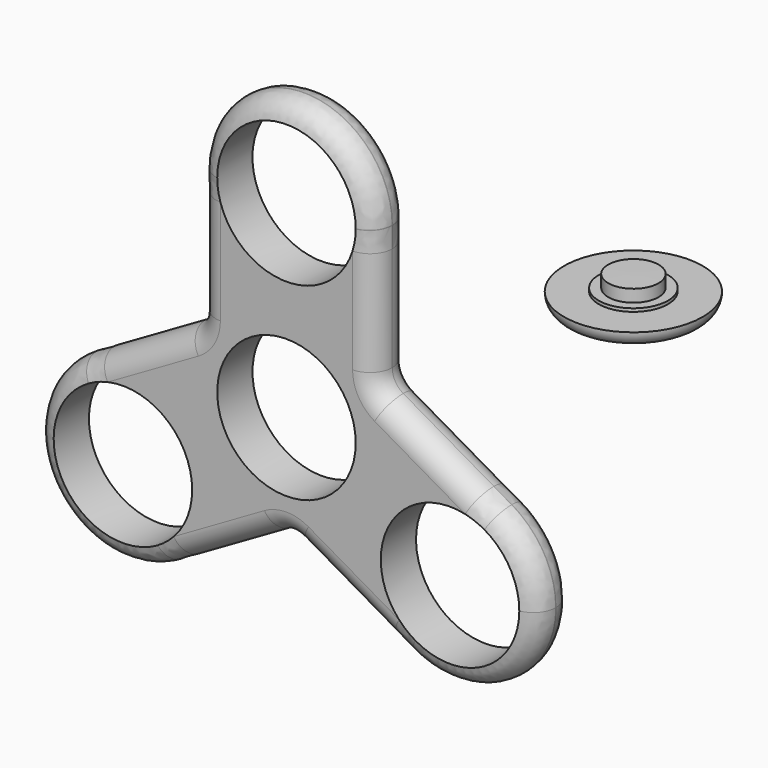
from build123d import *

# Parameters (mm, degrees)
F0_R     = 11
F1_DEPTH = 7
F2_R     = 3.49999
F5_R     = 2.49999


# Not quite as in the source:
# - a fillet or chamfer is up to 0.001 mm smaller than in the source, because OpenCascade refuses the exact size


with BuildPart() as f1:
    # F0 (on Front) → F1 (new body)
    with BuildSketch(Plane.XZ):
        with BuildLine():
            Line((14, 8.0829037687), (14, 30))
            ThreePointArc((14, 30), (0, 44), (-14, 30))
            Line((-14, 30), (-14, 8.0829037687))
            Line((-14, 8.0829037687), (-32.9807621135, -2.875644347))
            ThreePointArc((-32.9807621135, -2.875644347), (-38.1051177665, -22), (-18.9807621135, -27.124355653))
            Line((-18.9807621135, -27.124355653), (0, -16.1658075373))
            Line((0, -16.1658075373), (18.9807621135, -27.124355653))
            ThreePointArc((18.9807621135, -27.124355653), (38.1051177665, -22), (32.9807621135, -2.875644347))
            Line((32.9807621135, -2.875644347), (14, 8.0829037687))
        make_face()
        with Locations((-25.9807621135, -15)):
            Circle(F0_R, mode=Mode.SUBTRACT)
        with Locations((25.9807621135, -15)):
            Circle(F0_R, mode=Mode.SUBTRACT)
        Circle(F0_R, mode=Mode.SUBTRACT)
        with Locations((0, 30)):
            Circle(F0_R, mode=Mode.SUBTRACT)
    extrude(amount=F1_DEPTH)

    # F2 (radius 3.5 in the source; OpenCascade refuses exactly that, so slightly less here)
    f2_edges = [f1.edges().sort_by_distance(p)[0] for p in [
        (14, -3.5, 30),
        (-14, -3.5, 30),
        (0, 0, 44),
        (0, -7, 44),
        (32.980762, -3.5, -2.875644),
        (14, -3.5, 8.082904),
        (23.490381, 0, 2.60363),
        (23.490381, -7, 2.60363),
        (18.980762, -3.5, -27.124356),
        (38.105118, 0, -22),
        (38.105118, -7, -22),
        (-14, -3.5, 8.082904),
        (-14, 0, 19.041452),
        (-14, -7, 19.041452),
        (-32.980762, -3.5, -2.875644),
        (-23.490381, 0, 2.60363),
        (-23.490381, -7, 2.60363),
        (-18.980762, -3.5, -27.124356),
        (-38.105118, 0, -22),
        (-38.105118, -7, -22),
        (0, -3.5, -16.165808),
        (-9.490381, 0, -21.645082),
        (-9.490381, -7, -21.645082),
        (9.490381, 0, -21.645082),
        (9.490381, -7, -21.645082),
    ]]
    fillet(f2_edges, radius=F2_R)


with BuildPart() as f4:
    # F3 (on Front) → F4 (revolve)
    with BuildSketch(Plane.XZ):
        Polygon((53.5076283237, 33.3507540341), (49.5076283237, 33.399297446), (49.5076283237, 28.399297446), (60.5076283237, 28.399297446), (60.5076283237, 30.899297446), (55.0076283237, 30.899297446), (55.0076283237, 31.399297446), (53.5076283237, 31.399297446), align=None)
    revolve(axis=Axis((49.5076283237, 0, 30.899297446), (0, 0, -1)))

    # F5 (radius 2.5 in the source; OpenCascade refuses exactly that, so slightly less here)
    f5_edges = [f4.edges().sort_by_distance(p)[0] for p in [
        (38.507628, 0, 28.399297),
    ]]
    fillet(f5_edges, radius=F5_R)


solid = Compound([f1.part, f4.part])
